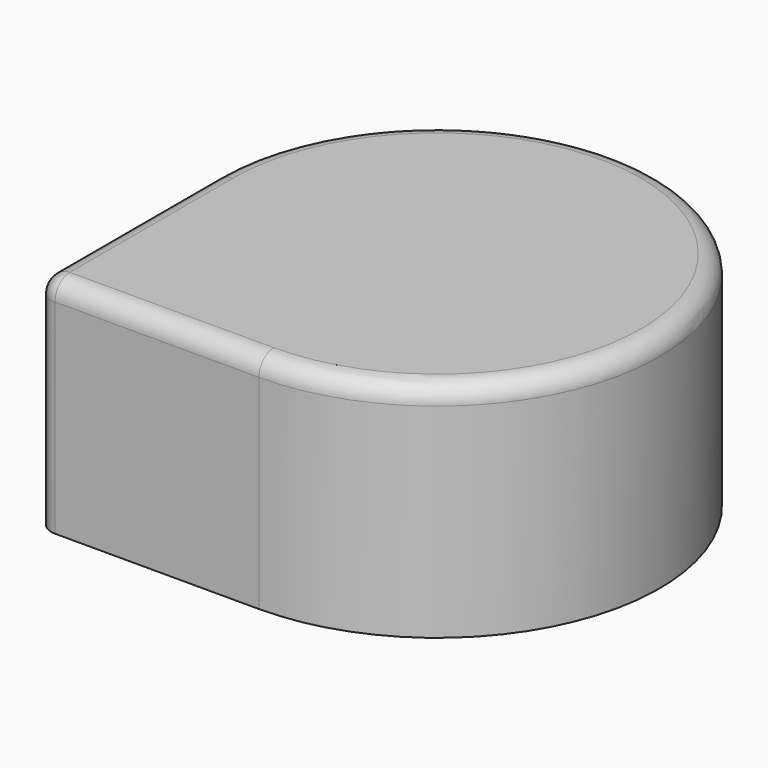
from build123d import *

# Parameters (mm, degrees)
F0_W     = 76.2
F0_H     = 76.2
F1_DEPTH = 76.2
F3_R     = 6.35
F4_T     = 6.35


# Not quite as in the source:
# - a shell that OpenCascade refuses in one call is made with other operations: the cavity is built on its own and cut out


with BuildPart() as f1:
    # F0 (on Front) → F1 (new body)
    with BuildSketch(Plane.XZ):
        with Locations((-38.1, 38.1)):
            Rectangle(F0_W, F0_H)
    extrude(amount=F1_DEPTH)

    # F0 (on Front) → F2 (revolve)
    with BuildSketch(Plane.XZ):
        with Locations((-38.1, 38.1)):
            Rectangle(F0_W, F0_H)
    revolve(axis=Axis((0, 0, 38.1), (0, 0, 1)))

    # F3
    f3_edges = [f1.edges().sort_by_distance(p)[0] for p in [
        (-76.2, -38.1, 76.2),
        (-76.2, -76.2, 38.1),
    ]]
    fillet(f3_edges, radius=F3_R)

    # F4: shell of thickness 6.35, made by hand


with BuildPart() as f4_core1:
    # F4_t2: copy of F1
    add(f1.part)

    # the walls: a layer under each face that stays
    f4_faces = [f4_core1.faces().sort_by_distance(p)[0] for p in [
        (-34.925, -76.2, 34.925),
        (53.8815367264, 53.8815367264, 34.925),
        (-76.2, -34.925, 34.925),
        (0, 0, 76.2),
    ]]
    thicken(f4_faces, amount=-F4_T, mode=Mode.SUBTRACT)


with BuildPart() as f1_1:
    add(f1.part)

    # what is left inside the walls is the cavity
    f4_cavity = [f4_core1.part.solids().sort_by_distance(p)[0] for p in [
        (49.346507, 49.346507, 46.566667),
    ]]
    add(f4_cavity, mode=Mode.SUBTRACT)


solid = f1_1.part
